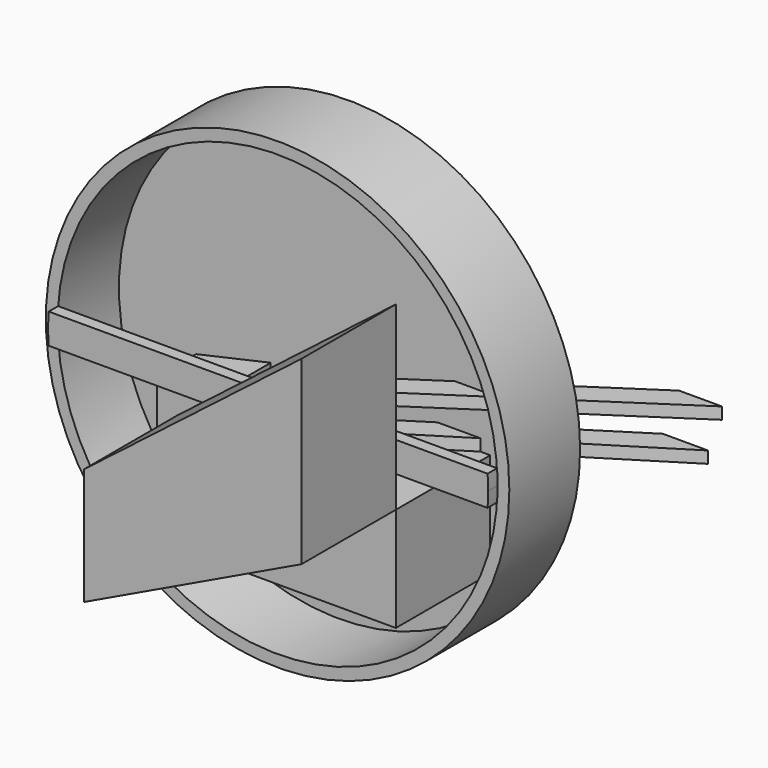
from build123d import *

# Parameters (mm, degrees)
F0_R      = 49.8968196512
F1_DEPTH  = 19.05
F2_T      = -2.54
F4_DEPTH  = 2.54
F6_DEPTH  = 2.54
F8_DEPTH  = 2.54
F12_DEPTH = 25.4
F14_DEPTH = 25.4
F16_DEPTH = 25.4


# Not quite as in the source:
# - a feature of the source that left no trace in its solid (it failed there, or was rolled back) is left out


with BuildPart() as f1:
    # F0 (on Front) → F1 (new body)
    with BuildSketch(Plane.XZ):
        Circle(F0_R)
    extrude(amount=F1_DEPTH)

    # F2
    f2_openings = [f1.faces().sort_by_distance(p)[0] for p in [
        (0, -19.05, 0),
    ]]
    offset(amount=F2_T, openings=f2_openings)

    # F5 (on face) → F6 (join)
    with BuildSketch(Plane.XY.offset(3.2400222074)):
        Polygon((56.5371960402, 18.3305814862), (0, -19.05), (9.2212408781, -19.05), (65.7584369183, 18.3305814862), align=None)
    extrude(amount=F6_DEPTH)

    # F7 (on face) → F8 (join)
    with BuildSketch(Plane(origin=(0, 0, -3.2400222074), x_dir=(1, 0, 0), z_dir=(0, 0, -1))):
        Polygon((4.062458419, 19.05), (-4.8034556786, 19.05), (53.3914454281, -17.8773459047), (63.1237998605, -17.8773459047), align=None)
    extrude(amount=F8_DEPTH)


with BuildPart() as f4:
    # F3 (on face) → F4 (new body)
    with BuildSketch(Plane.XZ.offset(19.05)):
        with BuildLine():
            Line((47.2458529775, 3.2400222074), (-47.2458529775, 3.2400222074))
            ThreePointArc((-47.2458529775, 3.2400222074), (-47.3568196512, 0), (-47.2458529775, -3.2400222074))
            Line((-47.2458529775, -3.2400222074), (47.2458529775, -3.2400222074))
            ThreePointArc((47.2458529775, -3.2400222074), (47.3290698525, -1.6209609424), (47.3568196512, 0))
            ThreePointArc((47.3568196512, 0), (47.3290698525, 1.6209609424), (47.2458529775, 3.2400222074))
        make_face()
    extrude(amount=F4_DEPTH)


with BuildPart() as f12:
    # F11 (on face) → F12 (new body)
    with BuildSketch(Plane(origin=(0, 0, -3.2400222074), x_dir=(1, 0, 0), z_dir=(0, 0, -1))):
        Polygon((-14.2288124189, 19.05), (-25.9999446571, 19.05), (-25.9999446571, 8.4945941344), (-14.2288124189, 3.1038702), align=None)
    extrude(amount=F12_DEPTH)


with BuildPart() as f14:
    # F13 (on face) → F14 (new body)
    with BuildSketch(Plane.XZ.offset(2.54)):
        Polygon((-14.2875006422, -5.7800222074), (-14.2875006422, -28.1940009445), (32.5755029917, -28.1940009445), (32.5755029917, -5.7800222074), (30.4684381424, -5.7800222074), (21.2151436476, -5.7800222074), align=None)
    extrude(amount=F14_DEPTH)

    # F15 (on face) → F16 (join)
    with BuildSketch(Plane.XZ.offset(27.94)):
        Polygon((-14.2875006422, -5.7800222074), (-14.2875006422, -28.1940009445), (32.5755029917, -5.7800222074), align=None)
        Polygon((-14.2875006422, -3.0480003916), (-14.2875006422, -5.7800222074), (32.5755029917, -5.7800222074), (32.5755029917, 33.1469997764), align=None)
    extrude(amount=F16_DEPTH)


solid = Compound([f1.part, f4.part, f12.part, f14.part])
